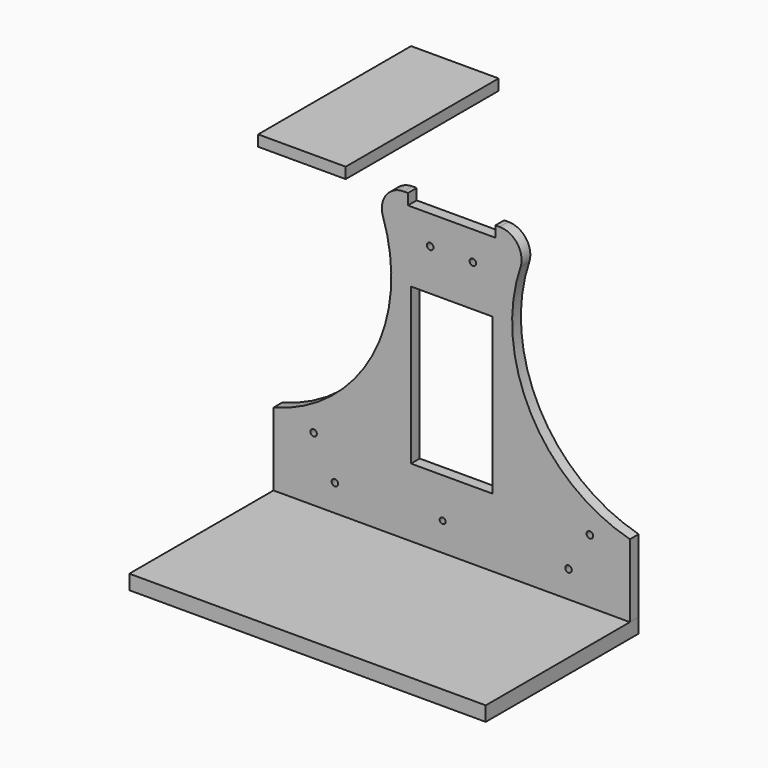
from build123d import *

# Parameters (mm, degrees)
F0_W     = 111.6156259179
F0_H     = 213.6525809765
F1_DEPTH = 15
F2_DEPTH = 262
F0_W_2   = 120
F0_H_2   = 15


# Not quite as in the source:
# - a feature names something its author has since deleted; it is built from what else it names


with BuildPart() as f1:
    # F0 (on Front) → F1 (new body)
    with BuildSketch(Plane.XZ):
        with BuildLine():
            Line((-244.2433449673, -200.5251348019), (-169.2433449673, -200.5251348019))
            Line((-169.2433449673, -200.5251348019), (169.2433449673, -200.5251348019))
            Line((169.2433449673, -200.5251348019), (244.2433449673, -200.5251348019))
            Line((244.2433449673, -200.5251348019), (244.2433449673, -100.5251348019))
            ThreePointArc((244.2433449673, -100.5251348019), (108.3515286863, 7.2241701212), (94.5992774336, 180.1038219864))
            ThreePointArc((94.5992774336, 180.1038219864), (89.6574888533, 206.3657523547), (65.7314252242, 218.2675900387))
            Line((65.7314252242, 218.2675900387), (60, 218.2675900387))
            Line((60, 218.2675900387), (60, 203.2777446508))
            Line((60, 203.2777446508), (39.5973048535, 203.2777446508))
            Line((39.5973048535, 203.2777446508), (-39.5973048535, 203.2777446508))
            Line((-39.5973048535, 203.2777446508), (-60, 203.2777446508))
            Line((-60, 203.2777446508), (-60, 218.2675900387))
            Line((-60, 218.2675900387), (-65.7314252242, 218.2675900387))
            ThreePointArc((-65.7314252242, 218.2675900387), (-89.6574888533, 206.3657523547), (-94.5992774336, 180.1038219864))
            ThreePointArc((-94.5992774336, 180.1038219864), (-108.3515286863, 7.2241701212), (-244.2433449673, -100.5251348019))
            Line((-244.2433449673, -100.5251348019), (-244.2433449673, -200.5251348019))
        make_face()
        Polygon((-160.320997, -168.251998), (-161.281004, -168.093993), (-162.184996, -167.733993), (-162.990003, -167.188003), (-163.658995, -166.481994), (-164.160993, -165.647994), (-164.471998, -164.725997), (-164.576994, -163.757995), (-164.471998, -162.791), (-164.160993, -161.869003), (-163.658995, -161.035003), (-162.990003, -160.328994), (-162.184996, -159.783004), (-161.281004, -159.423003), (-160.320997, -159.264999), (-159.348997, -159.317992), (-158.410993, -159.578002), (-157.552, -160.033996), (-156.809996, -160.664001), (-156.220991, -161.438995), (-155.813002, -162.322005), (-155.602995, -163.272002), (-155.602995, -164.244994), (-155.813002, -165.195007), (-156.220991, -166.078002), (-156.809996, -166.852996), (-157.552, -167.483001), (-158.378981, -167.921996), (-158.410993, -167.938995), (-159.348997, -168.199004), align=None, mode=Mode.SUBTRACT)
        Polygon((-192.251005, -109.666), (-191.445997, -109.120002), (-190.542005, -108.760001), (-189.581999, -108.601997), (-188.609999, -108.654998), (-187.671995, -108.915), (-186.813002, -109.371001), (-186.070997, -110.000999), (-185.481993, -110.776), (-185.074003, -111.659003), (-184.863996, -112.609), (-184.863996, -113.582), (-185.074003, -114.531997), (-185.481993, -115.415), (-186.070997, -116.190002), (-186.813002, -116.819999), (-187.671995, -117.276), (-188.609999, -117.536002), (-189.581999, -117.589004), (-190.542005, -117.430999), (-191.445997, -117.070998), (-192.251005, -116.525001), (-192.919996, -115.819), (-193.421995, -114.985), (-193.733, -114.063003), (-193.837995, -113.095), (-193.733, -112.127998), (-193.421995, -111.206001), (-192.919996, -110.372001), align=None, mode=Mode.SUBTRACT)
        with BuildLine():
            Line((-16.273001, -163.328994), (-16.577, -162.468993))
            Line((-16.577, -162.468993), (-16.3982734972, -162.4358947189))
            ThreePointArc((-16.3982734972, -162.4358947189), (-13.1824012189, -157.7582200028), (-8.5047265028, -160.9740922811))
            Line((-8.5047265028, -160.9740922811), (-8.326, -160.940994))
            Line((-8.326, -160.940994), (-8.302, -161.852996))
            Line((-8.302, -161.852996), (-8.476, -162.748))
            Line((-8.476, -162.748), (-8.838, -163.585006))
            Line((-8.838, -163.585006), (-9.373, -164.324004))
            Line((-9.373, -164.324004), (-9.570003543, -164.4993119854))
            ThreePointArc((-9.570003543, -164.4993119854), (-9.7831760908, -164.7035406724), (-10.0107826307, -164.8915490625))
            Line((-10.0107826307, -164.8915490625), (-10.054, -164.930007))
            Line((-10.054, -164.930007), (-10.0866973337, -164.9482859597))
            ThreePointArc((-10.0866973337, -164.9482859597), (-11.7188844595, -165.6514491376), (-13.4946947291, -165.580942724))
            Line((-13.4946947291, -165.580942724), (-13.536, -165.574996))
            Line((-13.536, -165.574996), (-13.5972583092, -165.5518721732))
            ThreePointArc((-13.5972583092, -165.5518721732), (-13.8690312333, -165.4602355471), (-14.1335667871, -165.3494260969))
            Line((-14.1335667871, -165.3494260969), (-14.389, -165.253005))
            Line((-14.389, -165.253005), (-15.152, -164.753997))
            Line((-15.152, -164.753997), (-15.79, -164.102996))
            Line((-15.79, -164.102996), (-16.273001, -163.328994))
        make_face(mode=Mode.SUBTRACT)
        Polygon((157.552001, -160.033996), (158.410994, -159.578002), (159.348997, -159.317992), (160.320997, -159.264999), (161.281004, -159.423003), (162.051908, -159.729995), (162.184996, -159.783004), (162.990003, -160.328994), (163.658995, -161.035003), (164.160993, -161.869003), (164.471998, -162.791), (164.576994, -163.757995), (164.471998, -164.725997), (164.160993, -165.647994), (163.658995, -166.481994), (162.990003, -167.188003), (162.184996, -167.733993), (161.281004, -168.093993), (160.320997, -168.251998), (159.348997, -168.199004), (158.410994, -167.938995), (157.552001, -167.483001), (156.809997, -166.852996), (156.220992, -166.078002), (155.813003, -165.195007), (155.602996, -164.244994), (155.602996, -163.272002), (155.813003, -162.322005), (156.220992, -161.438995), (156.809997, -160.664001), align=None, mode=Mode.SUBTRACT)
        Polygon((186.070997, -116.190002), (185.481993, -115.415), (185.074003, -114.531997), (184.863996, -113.582), (184.863996, -112.609), (185.074003, -111.659003), (185.481993, -110.776), (186.070997, -110.000999), (186.813002, -109.371001), (187.671995, -108.915), (188.609999, -108.654998), (189.581999, -108.601997), (190.542005, -108.760001), (191.445997, -109.120002), (192.251005, -109.666), (192.919996, -110.372001), (193.421995, -111.206001), (193.733, -112.127998), (193.837995, -113.095), (193.733, -114.063003), (193.421995, -114.985), (192.919996, -115.819), (192.251005, -116.525001), (191.445997, -117.070998), (190.542005, -117.430999), (189.581999, -117.589004), (188.609999, -117.536002), (187.671995, -117.276), (186.813002, -116.819999), align=None, mode=Mode.SUBTRACT)
        Rectangle(F0_W, F0_H, mode=Mode.SUBTRACT)
        Polygon((-31.742, 167.66699), (-30.851998, 168.059995), (-29.898, 168.251997), (-28.924998, 168.233991), (-27.979, 168.007993), (-27.103001, 167.583997), (-26.339001, 166.981001), (-25.723, 166.227995), (-25.282, 165.359998), (-25.039, 164.417997), (-25.004, 163.445997), (-25.179001, 162.488996), (-25.555, 161.591001), (-26.115, 160.796003), (-26.834, 160.13899), (-27.676001, 159.652998), (-28.603999, 159.358991), (-29.572999, 159.270994), (-30.537999, 159.393995), (-31.454999, 159.720991), (-32.278998, 160.238004), (-32.973998, 160.919004), (-33.505, 161.733991), (-33.848998, 162.645002), (-33.988997, 163.607999), (-33.918998, 164.578001), (-33.641997, 165.510999), (-33.171, 166.361997), (-32.526999, 167.093), align=None, mode=Mode.SUBTRACT)
        Polygon((31.672001, 160.132993), (31.022873, 159.757993), (30.829, 159.645994), (29.902, 159.352003), (28.933001, 159.26399), (27.966999, 159.386991), (27.051001, 159.714002), (26.226, 160.231001), (25.532, 160.912992), (25.000999, 161.727995), (24.657, 162.637998), (24.517, 163.600996), (24.587, 164.572004), (24.864, 165.503996), (25.334999, 166.356001), (25.979, 167.085996), (26.764, 167.660993), (27.653999, 168.052992), (28.608, 168.244993), (29.580999, 168.227995), (30.527, 168.001997), (31.403, 167.576994), (32.167, 166.973997), (32.783001, 166.221998), (33.223999, 165.354002), (33.466999, 164.412), (33.501999, 163.438993), (33.327, 162.481992), (32.951, 161.585004), (32.390999, 160.788999), align=None, mode=Mode.SUBTRACT)
        Polygon((169.2433449673, -200.5251348019), (-169.2433449673, -200.5251348019), (-244.2433449673, -200.5251348019), (-244.2433449673, -220.5251348019), (244.2433449673, -220.5251348019), (244.2433449673, -200.5251348019), align=None)
    extrude(amount=F1_DEPTH)


with BuildPart() as f2:
    # F0 (on Front) → F2 (new body)
    with BuildSketch(Plane.XZ):
        Polygon((169.2433449673, -200.5251348019), (-169.2433449673, -200.5251348019), (-244.2433449673, -200.5251348019), (-244.2433449673, -220.5251348019), (244.2433449673, -220.5251348019), (244.2433449673, -200.5251348019), align=None)
    extrude(amount=F2_DEPTH)


with BuildPart() as f2b:
    # F0 (on Front) → F2, piece 2 (new body)
    with BuildSketch(Plane.XZ):
        with Locations((-7.6870495081, 379.4182908535)):
            Rectangle(F0_W_2, F0_H_2)
    extrude(amount=F2_DEPTH)


solid = Compound([f1.part, f2.part, f2b.part])
